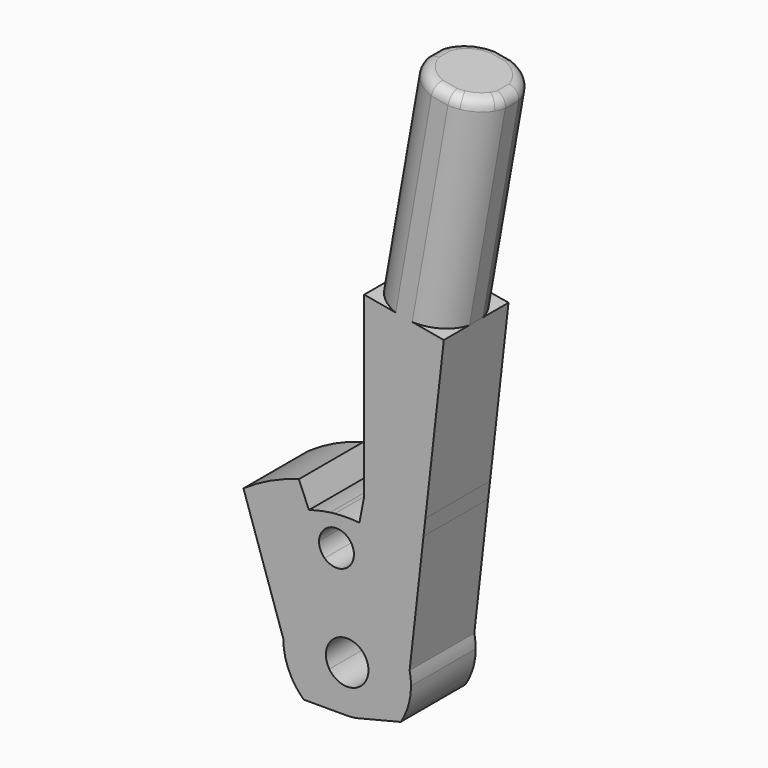
from build123d import *

# Parameters (mm, degrees)
F1_DEPTH     = 9.5
F3_DEPTH     = 25.4
F4_T3_ANGLE  = 141.5409724071
F4_T6_ANGLE  = 141.5409724071
F4_T9_ANGLE  = 141.5409724071
F4_T12_ANGLE = 141.5409724071
F4_T15_DEPTH = 8.3234051383
F4_T18_DEPTH = 8.3234051383
F4_T21_DEPTH = 8.3234051383
F4_T24_DEPTH = 8.3234051383


# Not quite as in the source:
# - a fillet or chamfer that OpenCascade refuses, or shapes differently, is made with other operations: its cross-section is extruded or revolved along the edge and cut away or added
# - a feature names something its author has since deleted; it is built from what else it names


with BuildPart() as f1:
    # F0 (on Front) → F1 (new body)
    with BuildSketch(Plane.XZ):
        with BuildLine():
            ThreePointArc((-6.278127268, -4.1030620281), (-5.7312935841, -4.8375896739), (-5.0990195136, -5.5))
            Line((-5.0990195136, -5.5), (0, -5.5))
            ThreePointArc((0, -5.5), (-0.6705781, -5.4589673943), (-1.3311505394, -5.3364818224))
            Line((-1.3311505394, -5.3364818224), (-6.2774946566, -4.1026485857))
            Line((-6.2774946566, -4.1026485857), (-6.278127268, -4.1030620281))
        make_face()
        with BuildLine():
            ThreePointArc((-1.3311505394, -5.3364818224), (-0.6705781, -5.4589673943), (0, -5.5))
            ThreePointArc((0, -5.5), (0.6702813887, -5.459003834), (1.3305704258, -5.3366264945))
            ThreePointArc((1.3305704258, -5.3366264945), (2.6173443749, -4.8373038382), (3.7392809766, -4.0333333333))
            Line((3.7392809766, -4.0333333333), (3.2448291178, -3.4999984017))
            Line((3.2448291178, -3.4999984017), (-4.2426420057, -3.4999984017))
            ThreePointArc((-4.2426420057, -3.4999984017), (-2.9342731081, -4.6518857818), (-1.3311505394, -5.3364818224))
        make_face()
        with BuildLine():
            Line((5.3553749013, -3.4999984017), (6.278127268, -4.1030620281))
            ThreePointArc((6.278127268, -4.1030620281), (6.4627269717, -3.8056747219), (6.6332504241, -3.4999984017))
            Line((6.6332504241, -3.4999984017), (5.3553749013, -3.4999984017))
        make_face()
        with BuildLine():
            Line((4.2684615244, -4.6041279743), (6.278127268, -4.1030620281))
            Line((6.278127268, -4.1030620281), (5.3553749013, -3.4999984017))
            Line((5.3553749013, -3.4999984017), (4.2426420057, -3.4999984017))
            ThreePointArc((4.2426420057, -3.4999984017), (3.9998606427, -3.7750648788), (3.7392809766, -4.0333333333))
            Line((3.7392809766, -4.0333333333), (4.2684615244, -4.6041279743))
        make_face()
        with BuildLine():
            Line((1.3305704258, -5.3366264945), (4.2684615244, -4.6041279743))
            Line((4.2684615244, -4.6041279743), (3.7392809766, -4.0333333333))
            ThreePointArc((3.7392809766, -4.0333333333), (2.6173443749, -4.8373038382), (1.3305704258, -5.3366264945))
        make_face()
        with BuildLine():
            Line((5.3553749013, -3.4999984017), (6.6332504241, -3.4999984017))
            ThreePointArc((6.6332504241, -3.4999984017), (7.2800885359, -1.8028618665), (7.5, 0))
            ThreePointArc((7.5, 0), (7.4589142153, 0.7839634745), (7.3361070055, 1.5593376811))
            Line((7.3361070055, 1.5593376811), (0, 7.5))
            ThreePointArc((0, 7.5), (-0.7821825791, 7.45910118), (-1.5558343996, 7.3368507768))
            ThreePointArc((-1.5558343996, 7.3368507768), (-5.8274676317, 4.7212944201), (-7.5, 0))
            ThreePointArc((-7.5, 0), (-7.2800885359, -1.8028618665), (-6.6332504241, -3.4999984017))
            Line((-6.6332504241, -3.4999984017), (-5.3553749013, -3.4999984017))
            Line((-5.3553749013, -3.4999984017), (-2.0927090893, -1.3676873427))
            ThreePointArc((-2.0927090893, -1.3676873427), (-0.7135219957, 2.3960146831), (2.5, 0))
            ThreePointArc((2.5, 0), (2.3960146831, -0.7135219957), (2.0927090893, -1.3676873427))
            Line((2.0927090893, -1.3676873427), (5.3553749013, -3.4999984017))
        make_face()
        with BuildLine():
            ThreePointArc((-6.6332504241, -3.4999984017), (-6.4629338114, -3.8053234487), (-6.278573257, -4.1023795359))
            Line((-6.278573257, -4.1023795359), (-6.2774946566, -4.1026485857))
            Line((-6.2774946566, -4.1026485857), (-5.3553749013, -3.4999984017))
            Line((-5.3553749013, -3.4999984017), (-6.6332504241, -3.4999984017))
        make_face()
        with BuildLine():
            Line((-5.3553749013, -3.4999984017), (-6.2774946566, -4.1026485857))
            Line((-6.2774946566, -4.1026485857), (-1.3311505394, -5.3364818224))
            ThreePointArc((-1.3311505394, -5.3364818224), (-2.9342731081, -4.6518857818), (-4.2426420057, -3.4999984017))
            Line((-4.2426420057, -3.4999984017), (-5.3553749013, -3.4999984017))
        make_face()
        with BuildLine():
            Line((4.2426420057, -3.4999984017), (5.3553749013, -3.4999984017))
            Line((5.3553749013, -3.4999984017), (2.0927090893, -1.3676873427))
            ThreePointArc((2.0927090893, -1.3676873427), (1.9104311947, -1.6125298913), (1.6996731712, -1.8333333333))
            Line((1.6996731712, -1.8333333333), (3.2448291178, -3.4999984017))
            Line((3.2448291178, -3.4999984017), (4.2426420057, -3.4999984017))
        make_face()
        with BuildLine():
            Line((3.2448291178, -3.4999984017), (3.7392809766, -4.0333333333))
            ThreePointArc((3.7392809766, -4.0333333333), (3.9998606427, -3.7750648788), (4.2426420057, -3.4999984017))
            Line((4.2426420057, -3.4999984017), (3.2448291178, -3.4999984017))
        make_face()
        with BuildLine():
            ThreePointArc((2, 17.8124786447), (5.562192945, 17.1823042647), (8.9673456279, 15.9611271549))
            Line((8.9673456279, 15.9611271549), (9.1869547449, 17.9))
            Line((9.1869547449, 17.9), (2, 17.9))
            Line((2, 17.9), (2, 17.8124786447))
        make_face()
        with BuildLine():
            Line((7.3361070055, 1.5593376811), (8.9673456279, 15.9611271549))
            ThreePointArc((8.9673456279, 15.9611271549), (5.562192945, 17.1823042647), (2, 17.8124786447))
            Line((2, 17.8124786447), (2, 14.8660687473))
            ThreePointArc((2, 14.8660687473), (1.7208485958, 14.9009623887), (1.4410918883, 14.9306146615))
            Line((1.4410918883, 14.9306146615), (0.7907929481, 11.5775176947))
            ThreePointArc((0.7907929481, 11.5775176947), (0.7947016791, 11.5045182456), (0.796005142, 11.431425847))
            ThreePointArc((0.796005142, 11.431425847), (0.74331089, 10.9696144689), (0.5879370942, 10.531544364))
            Line((0.5879370942, 10.531544364), (0, 7.5))
            ThreePointArc((0, 7.5), (4.7199029329, 5.8285947109), (7.3361070055, 1.5593376811))
        make_face()
        with BuildLine():
            Line((-2.0927090893, -1.3676873427), (-5.3553749013, -3.4999984017))
            Line((-5.3553749013, -3.4999984017), (-4.2426420057, -3.4999984017))
            Line((-4.2426420057, -3.4999984017), (3.2448291178, -3.4999984017))
            Line((3.2448291178, -3.4999984017), (1.6996731712, -1.8333333333))
            ThreePointArc((1.6996731712, -1.8333333333), (-0.3046733585, -2.4813653791), (-2.0927090893, -1.3676873427))
        make_face()
        Polygon((2, 17.9), (9.1869547449, 17.9), (11.3556736536, 37.0470657463), (2, 38.6967234342), align=None)
        with BuildLine():
            Line((0, 7.5), (7.3361070055, 1.5593376811))
            ThreePointArc((7.3361070055, 1.5593376811), (4.7199029329, 5.8285947109), (0, 7.5))
        make_face()
        with BuildLine():
            Line((2, 14.8660687473), (2, 17.8124786447))
            Line((2, 17.8124786447), (1.4410918883, 14.9306146615))
            ThreePointArc((1.4410918883, 14.9306146615), (1.7208485958, 14.9009623887), (2, 14.8660687473))
        make_face()
        with BuildLine():
            Line((-12.1821134163, 14.0479597482), (-7.5, 0))
            ThreePointArc((-7.5, 0), (-5.8274676317, 4.7212944201), (-1.5558343996, 7.3368507768))
            Line((-1.5558343996, 7.3368507768), (-2.6466676169, 9.9271111902))
            ThreePointArc((-2.6466676169, 9.9271111902), (-3.1432959169, 10.6357867901), (-3.3032618841, 11.4862405888))
            Line((-3.3032618841, 11.4862405888), (-4.492973918, 14.3112957265))
            Line((-4.492973918, 14.3112957265), (-5.6739843882, 17.1156883874))
            ThreePointArc((-5.6739843882, 17.1156883874), (-9.0578982258, 15.8572969832), (-12.1821134163, 14.0479597482))
        make_face()
        with BuildLine():
            Line((-0.4013869334, 9.5671405344), (0, 7.5))
            Line((0, 7.5), (0.5879370942, 10.531544364))
            ThreePointArc((0.5879370942, 10.531544364), (0.1769680952, 9.9634868066), (-0.4013869334, 9.5671405344))
        make_face()
        with BuildLine():
            ThreePointArc((-1.5558343996, 7.3368507768), (-0.7821825791, 7.45910118), (0, 7.5))
            Line((0, 7.5), (-0.4013869334, 9.5671405344))
            ThreePointArc((-0.4013869334, 9.5671405344), (-1.5785133083, 9.4072747224), (-2.6466676169, 9.9271111902))
            Line((-2.6466676169, 9.9271111902), (-1.5558343996, 7.3368507768))
        make_face()
        with BuildLine():
            Line((0.7907929481, 11.5775176947), (1.4410918883, 14.9306146615))
            ThreePointArc((1.4410918883, 14.9306146615), (-0.0008616205, 14.9999999753), (-1.4428071487, 14.9304490064))
            Line((-1.4428071487, 14.9304490064), (-1.1610336493, 13.4793170096))
            ThreePointArc((-1.1610336493, 13.4793170096), (0.1766353776, 12.8996891507), (0.7907929481, 11.5775176947))
        make_face()
        with BuildLine():
            Line((-1.1610336493, 13.4793170096), (-1.4428071487, 14.9304490064))
            ThreePointArc((-1.4428071487, 14.9304490064), (-1.7217045246, 14.9008635162), (-2, 14.8660687473))
            ThreePointArc((-2, 14.8660687473), (-3.2583156463, 14.6418366044), (-4.492973918, 14.3112957265))
            Line((-4.492973918, 14.3112957265), (-3.3032618841, 11.4862405888))
            ThreePointArc((-3.3032618841, 11.4862405888), (-2.6503728575, 12.9323017521), (-1.1610336493, 13.4793170096))
        make_face()
    extrude(amount=F1_DEPTH)

    # F2 (on face) → F3 (join)
    with BuildSketch(Plane(origin=(6.6778368268, 0, 37.8718945902), x_dir=(0.984807753, 0, -0.1736481777), z_dir=(0.1736481777, 0, 0.984807753))):
        with BuildLine():
            Line((4.75, -5.7367025692), (4.75, -3.7632974308))
            ThreePointArc((4.75, -3.7632974308), (3.4304578382, -1.3195421618), (0.9867025692, 0))
            Line((0.9867025692, 0), (-0.9867025692, 0))
            ThreePointArc((-0.9867025692, 0), (-3.4304578382, -1.3195421618), (-4.75, -3.7632974308))
            Line((-4.75, -3.7632974308), (-4.75, -5.7367025692))
            ThreePointArc((-4.75, -5.7367025692), (-3.4304578382, -8.1804578382), (-0.9867025692, -9.5))
            Line((-0.9867025692, -9.5), (0.9867025692, -9.5))
            ThreePointArc((0.9867025692, -9.5), (3.4304578382, -8.1804578382), (4.75, -5.7367025692))
        make_face()
    extrude(amount=F3_DEPTH)

    # F4: fillet of radius 1.27 on 8 edges, made by hand


with BuildPart() as f4_tool1:
    # F4_s2 → F4_t3 (revolve)
    with BuildSketch(Plane(origin=(-1.8314973588, -3.8521427254, 0.3229423995), x_dir=(0.9031202932, -0.4293876291, 0), z_dir=(-0.428162184, -0.9005428451, 0.0754965452))):
        with BuildLine():
            ThreePointArc((16.6460437024, 60.7270239449), (16.4195050257, 61.6722726811), (15.5909262, 62.1804774378))
            Line((15.5909262, 62.1804774378), (16.8452116977, 61.9813094426))
            Line((16.8452116977, 61.9813094426), (16.6460437024, 60.7270239449))
        make_face()
    revolve(axis=Axis((11.0885005395, -4.75, 62.8860115168), (0.1736481777, 0, 0.984807753)), revolution_arc=F4_T3_ANGLE)


with BuildPart() as f4_tool4:
    # F4_s5 → F4_t6 (revolve)
    with BuildSketch(Plane(origin=(-1.8314973588, -3.8521427254, 0.3229423995), x_dir=(-0.9031202932, 0.4293876291, 0), z_dir=(0.428162184, 0.9005428451, -0.0754965452))):
        with BuildLine():
            ThreePointArc((-8.5167559932, 63.3037849312), (-7.571507257, 63.0772462545), (-7.0633025002, 62.2486674288))
            Line((-7.0633025002, 62.2486674288), (-7.2624704955, 63.5029529265))
            Line((-7.2624704955, 63.5029529265), (-8.5167559932, 63.3037849312))
        make_face()
    revolve(axis=Axis((11.0885005395, -4.75, 62.8860115168), (0.1736481777, 0, 0.984807753)), revolution_arc=F4_T6_ANGLE)


with BuildPart() as f4_tool7:
    # F4_s8 → F4_t9 (revolve)
    with BuildSketch(Plane(origin=(1.8314973588, -0.8978572746, -0.3229423995), x_dir=(-0.4401826931, -0.897908234, 0), z_dir=(-0.8868615758, 0.4347672758, 0.156377624))):
        with BuildLine():
            ThreePointArc((2.9550204056, 64.2700294569), (3.8788513484, 63.9677856244), (4.3183798092, 63.1008198364))
            Line((4.3183798092, 63.1008198364), (4.2213049176, 64.3671043485))
            Line((4.2213049176, 64.3671043485), (2.9550204056, 64.2700294569))
        make_face()
    revolve(axis=Axis((11.0885005395, -4.75, 62.8860115168), (0.1736481777, 0, 0.984807753)), revolution_arc=F4_T9_ANGLE)


with BuildPart() as f4_tool10:
    # F4_s11 → F4_t12 (revolve)
    with BuildSketch(Plane(origin=(1.8314973588, -0.8978572746, -0.3229423995), x_dir=(0.4401826931, 0.897908234, 0), z_dir=(0.8868615758, -0.4347672758, -0.156377624))):
        with BuildLine():
            ThreePointArc((5.3560338628, 62.3591676648), (5.0537900302, 63.2829986077), (4.1868242423, 63.7225270684))
            Line((4.1868242423, 63.7225270684), (5.4531087544, 63.6254521769))
            Line((5.4531087544, 63.6254521769), (5.3560338628, 62.3591676648))
        make_face()
    revolve(axis=Axis((11.0885005395, -4.75, 62.8860115168), (0.1736481777, 0, 0.984807753)), revolution_arc=F4_T12_ANGLE)


with BuildPart() as f4_tool13:
    # F4_s14 → F4_t15 (new body)
    with BuildSketch(Plane.XZ.offset(0.5882974308)):
        with BuildLine():
            ThreePointArc((7.6613695591, 63.490307175), (6.7123942993, 63.279924425), (6.1901305271, 62.4601345144))
            Line((6.1901305271, 62.4601345144), (6.4106637127, 63.7108403607))
            Line((6.4106637127, 63.7108403607), (7.6613695591, 63.490307175))
        make_face()
    extrude(amount=F4_T15_DEPTH)


with BuildPart() as f4_tool16:
    # F4_s17 → F4_t18 (new body)
    with BuildSketch(Plane(origin=(4.0984769558, 0, -0.7226720671), x_dir=(0, 1, 0), z_dir=(-0.984807753, 0, 0.1736481777))):
        with BuildLine():
            ThreePointArc((0, -62.5861296095), (-0.3719743879, -63.4841552216), (-1.27, -63.8561296095))
            Line((-1.27, -63.8561296095), (0, -63.8561296095))
            Line((0, -63.8561296095), (0, -62.5861296095))
        make_face()
    extrude(amount=F4_T18_DEPTH)


with BuildPart() as f4_tool19:
    # F4_s20 → F4_t21 (new body)
    with BuildSketch(Plane(origin=(-4.0984769558, 0, 0.7226720671), x_dir=(0, 1, 0), z_dir=(0.984807753, 0, -0.1736481777))):
        with BuildLine():
            ThreePointArc((-9.5, 62.5861296095), (-9.1280256121, 63.4841552216), (-8.23, 63.8561296095))
            Line((-8.23, 63.8561296095), (-9.5, 63.8561296095))
            Line((-9.5, 63.8561296095), (-9.5, 62.5861296095))
        make_face()
    extrude(amount=F4_T21_DEPTH)


with BuildPart() as f4_tool22:
    # F4_s23 → F4_t24 (new body)
    with BuildSketch(Plane.XZ.offset(8.9117025692)):
        with BuildLine():
            ThreePointArc((15.5458041807, 60.8104768265), (15.3354214306, 61.7594520863), (14.51563152, 62.2817158585))
            Line((14.51563152, 62.2817158585), (15.7663373664, 62.0611826728))
            Line((15.7663373664, 62.0611826728), (15.5458041807, 60.8104768265))
        make_face()
    extrude(amount=-F4_T24_DEPTH)


with BuildPart() as f1_1:
    add(f1.part)

    # F4_t25: cut F4_tool1, F4_tool4, F4_tool7, F4_tool10, F4_tool13, F4_tool16, F4_tool19, F4_tool22
    add([f4_tool1.part, f4_tool4.part, f4_tool7.part, f4_tool10.part, f4_tool13.part, f4_tool16.part, f4_tool19.part, f4_tool22.part], mode=Mode.SUBTRACT)


solid = f1_1.part
